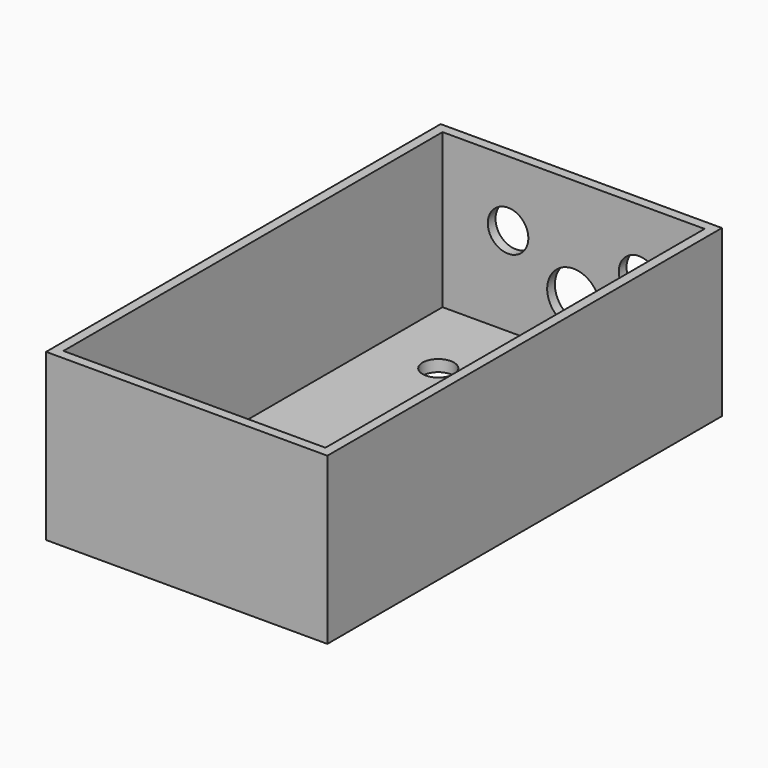
from build123d import *

# Parameters (mm, degrees)
F0_W         = 73
F0_H         = 128
F1_DEPTH     = 43
F2_W         = 68
F2_H         = 123
F3_DEPTH     = 40
F4_R         = 4.071875
F4_R_2       = 6.35
F4_R_3       = 3.675
F5_DEPTH     = 25
F6_R         = 6.85
F6_R_2       = 5.2625
F7_DEPTH     = 25
F9_TEXT_SIZE = 6.9444444444
F10_DEPTH    = 1.5


# Not quite as in the source:
# - Text() gives the source's letters only with a copy of the font that has no kerning and outlines rounded to 1/6400 em; it was checked with that copy


with BuildPart() as f1:
    # F0 (on Top) → F1 (new body)
    with BuildSketch(Plane.XY):
        Rectangle(F0_W, F0_H)
    extrude(amount=F1_DEPTH)

    # F2 (on face) → F3 (cut)
    with BuildSketch(Plane.XY.offset(43)):
        Rectangle(F2_W, F2_H)
    extrude(amount=-F3_DEPTH, mode=Mode.SUBTRACT)

    # F4 (on face) → F5 (cut)
    with BuildSketch(Plane.XY.offset(3)):
        with Locations((-17.9119046929, 40)):
            Circle(F4_R)
        with Locations((0, 40)):
            Circle(F4_R)
        with Locations((17.9119046929, 40)):
            Circle(F4_R)
        with Locations((0, -33)):
            Circle(F4_R_2)
        with Locations((8.9559523465, 15)):
            Circle(F4_R_3)
        Circle(F4_R_3)
    extrude(amount=-F5_DEPTH, mode=Mode.SUBTRACT)

    # F6 (on face) → F7 (cut)
    with BuildSketch(Plane.XZ.offset(-61.5)):
        with Locations((0, 16)):
            Circle(F6_R)
        with Locations((17, 26)):
            Circle(F6_R_2)
        with Locations((-17, 26)):
            Circle(F6_R_2)
    extrude(amount=-F7_DEPTH, mode=Mode.SUBTRACT)

    # F9 (on face) → F10 (cut)
    with BuildSketch(Plane(origin=(0, 0, 0), x_dir=(1, 0, 0), z_dir=(0, 0, -1))):
        with Locations(Location((29.3945663914, -53), (0, 0, 180))):
            Text('VOL', F9_TEXT_SIZE, font='Open Sans', font_style=FontStyle.BOLD, text_align=(TextAlign.LEFT, TextAlign.BOTTOM))
        with Locations(Location((9.5616319444, -53), (0, 0, 180))):
            Text('TONE', F9_TEXT_SIZE, font='Open Sans', font_style=FontStyle.BOLD, text_align=(TextAlign.LEFT, TextAlign.BOTTOM))
        with Locations(Location((-11.8034205581, -53), (0, 0, 180))):
            Text('GAIN', F9_TEXT_SIZE, font='Open Sans', font_style=FontStyle.BOLD, text_align=(TextAlign.LEFT, TextAlign.BOTTOM))
    extrude(amount=-F10_DEPTH, mode=Mode.SUBTRACT)


solid = f1.part
